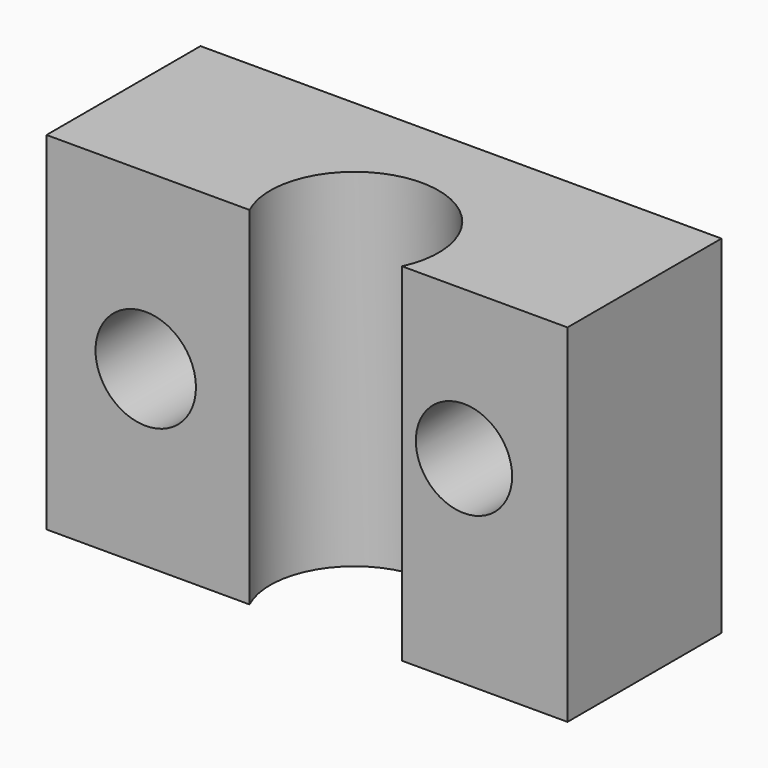
from build123d import *

# Parameters (mm, degrees)
F0_W       = 137.4987065792
F0_H       = 91.6657298803
F1_DEPTH   = 76.2
F3_R       = 34.4698963813
F4_DEPTH   = 76.2
F5_R       = 33.2776122009
F1_FACE1_W = 137.4987065792
F1_FACE1_H = 91.6657298803
F6_DEPTH   = 25.4
F7_R       = 29.7028077698
F8_DEPTH   = 25.4
F9_R       = 24.8229893925
F10_DEPTH  = 25.4
F11_R      = 22.2267461951
F12_DEPTH  = 127
F13_R      = 13.2555629358
F14_DEPTH  = 127
F15_R      = 12.3283716693
F16_DEPTH  = 127
F17_R      = 13.7331139198
F19_DEPTH  = 127
F21_R      = 15.0922963459
F22_DEPTH  = 127
F23_R      = 12.709116002
F24_DEPTH  = 152.4


# Not quite as in the source:
# - a feature of the source that left no trace in its solid (it failed there, or was rolled back) is left out


with BuildPart() as f1:
    # F0 (on Front) → F1 (new body)
    with BuildSketch(Plane.XZ):
        Rectangle(F0_W, F0_H)
    extrude(amount=F1_DEPTH)

    # F3 (on Front) → F4 (cut)
    with BuildSketch(Plane.XZ):
        with Locations((0, 31.9152921438)):
            Circle(F3_R)
    extrude(amount=-F4_DEPTH, mode=Mode.SUBTRACT)

    # F5 (on Front) + F1_face1 (on face) → F6 (cut)
    with BuildSketch(Plane.XZ):
        with Locations((0, 32.8243151307)):
            Circle(F5_R)
    with BuildSketch(Plane.XZ.offset(76.2)):
        Rectangle(F1_FACE1_W, F1_FACE1_H)
    extrude(amount=-F6_DEPTH, mode=Mode.SUBTRACT)

    # F7 (on Front) → F8 (cut)
    with BuildSketch(Plane.XZ):
        with Locations((0, 34.5415323973)):
            Circle(F7_R)
    extrude(amount=-F8_DEPTH, mode=Mode.SUBTRACT)

    # F9 (on Front) → F10 (cut)
    with BuildSketch(Plane.XZ):
        with Locations((0, 21.1320593953)):
            Circle(F9_R)
    extrude(amount=-F10_DEPTH, mode=Mode.SUBTRACT)

    # F11 (on face) → F12 (cut)
    with BuildSketch(Plane.XY.offset(45.8328649402)):
        with Locations((4.9597388133, -41.3516201079)):
            Circle(F11_R)
    extrude(amount=-F12_DEPTH, mode=Mode.SUBTRACT)

    # F13 (on face) → F14 (cut)
    with BuildSketch(Plane.XZ.offset(50.8)):
        with Locations((-42.5670817494, 0)):
            Circle(F13_R)
    extrude(amount=-F14_DEPTH, mode=Mode.SUBTRACT)

    # F15 (on Front) → F16 (cut)
    with BuildSketch(Plane.XZ):
        with Locations((51.0331951082, 0)):
            Circle(F15_R)
    extrude(amount=-F16_DEPTH, mode=Mode.SUBTRACT)

    # F17 (on Front) → F19 (cut)
    with BuildSketch(Plane.XZ):
        with Locations((48.1030344963, 0)):
            Circle(F17_R)
    extrude(amount=-F19_DEPTH, mode=Mode.SUBTRACT)

    # F21 (on Front) → F22 (cut)
    with BuildSketch(Plane.XZ):
        with Locations((40.081076324, 0)):
            Circle(F21_R)
    extrude(amount=-F22_DEPTH, mode=Mode.SUBTRACT)

    # F23 (on Front) → F24 (cut)
    with BuildSketch(Plane.XZ):
        with Locations((41.4244011045, 6.4881131984)):
            Circle(F23_R)
    extrude(amount=F24_DEPTH, mode=Mode.SUBTRACT)


solid = f1.part
